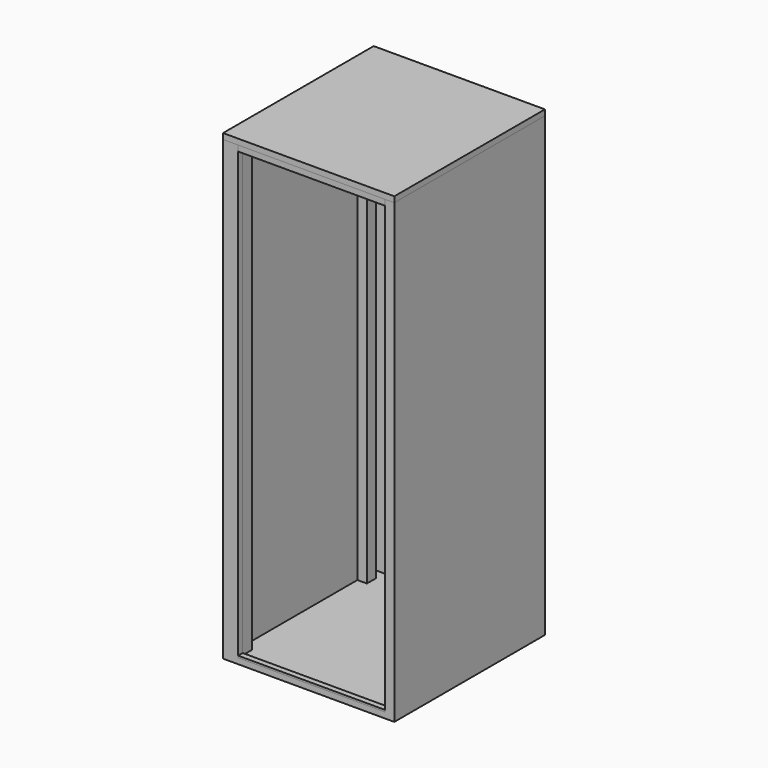
from build123d import *

# Parameters (mm, degrees)
F1_DEPTH  = 1514.475
F3_DEPTH  = 19.05
F5_DEPTH  = 19.05
F6_W      = 492.125
F6_H      = 6.35
F7_DEPTH  = 19.05
F8_W      = 492.125
F8_H      = 19.05
F9_DEPTH  = 19.05
F10_W     = 12.7
F10_H     = 38.1
F11_DEPTH = 1514.475
F10_W_2   = 31.75


# Not quite as in the source:
# - a feature names something its author has since deleted; it is built from what else it names


with BuildPart() as f1:
    # F0 (on Top) → F1 (new body)
    with BuildSketch(Plane.XY):
        Polygon((0, 631.825), (0, 0), (50.8, 0), (50.8, 19.05), (19.05, 19.05), (19.05, 612.775), (555.625, 612.775), (555.625, 19.05), (542.925, 19.05), (542.925, 0), (574.675, 0), (574.675, 631.825), align=None)
    extrude(amount=F1_DEPTH)

    # F4 (on face) → F5 (join)
    with BuildSketch(Plane(origin=(0, 0, 0), x_dir=(1, 0, 0), z_dir=(0, 0, -1))):
        Polygon((542.925, 0), (50.8, 0), (50.8, -19.05), (19.05, -19.05), (19.05, -612.775), (555.625, -612.775), (555.625, -19.05), (542.925, -19.05), align=None)
        Polygon((50.8, 0), (0, 0), (0, -631.825), (574.675, -631.825), (574.675, 0), (542.925, 0), (542.925, -19.05), (555.625, -19.05), (555.625, -612.775), (19.05, -612.775), (19.05, -19.05), (50.8, -19.05), align=None)
    extrude(amount=F5_DEPTH)


with BuildPart() as f3:
    # F2 (on face) → F3 (new body)
    with BuildSketch(Plane.XY.offset(1514.475)):
        Polygon((574.675, 631.825), (0, 631.825), (0, 0), (50.8, 0), (50.8, 19.05), (19.05, 19.05), (19.05, 612.775), (555.625, 612.775), (555.625, 19.05), (542.925, 19.05), (542.925, 0), (574.675, 0), align=None)
        Polygon((50.8, 19.05), (50.8, 0), (542.925, 0), (542.925, 19.05), (555.625, 19.05), (555.625, 612.775), (19.05, 612.775), (19.05, 19.05), align=None)
    extrude(amount=F3_DEPTH)


with BuildPart() as f7:
    # F6 (on face) → F7 (new body)
    with BuildSketch(Plane.XZ):
        with Locations((296.8625, 3.175)):
            Rectangle(F6_W, F6_H)
    extrude(amount=-F7_DEPTH)


with BuildPart() as f9:
    # F8 (on face) → F9 (new body)
    with BuildSketch(Plane.XZ):
        with Locations((296.8625, 1504.95)):
            Rectangle(F8_W, F8_H)
    extrude(amount=-F9_DEPTH)


with BuildPart() as f11:
    # F10 (on face) → F11 (new body, through all)
    with BuildSketch(Plane.XY):
        with Locations((549.275, 593.725)):
            Rectangle(F10_W, F10_H)
    extrude(amount=F11_DEPTH)


with BuildPart() as f11b:
    # F10 (on face) → F11, piece 2 (new body, through all)
    with BuildSketch(Plane.XY):
        with Locations((549.275, 38.1)):
            Rectangle(F10_W, F10_H)
    extrude(amount=F11_DEPTH)


with BuildPart() as f11c:
    # F10 (on face) → F11, piece 3 (new body, through all)
    with BuildSketch(Plane.XY):
        with Locations((34.925, 38.1)):
            Rectangle(F10_W_2, F10_H)
    extrude(amount=F11_DEPTH)


with BuildPart() as f11d:
    # F10 (on face) → F11, piece 4 (new body, through all)
    with BuildSketch(Plane.XY):
        with Locations((34.925, 558.8)):
            Rectangle(F10_W_2, F10_H)
    extrude(amount=F11_DEPTH)


solid = Compound([f1.part, f3.part, f7.part, f9.part, f11.part, f11b.part, f11c.part, f11d.part])
